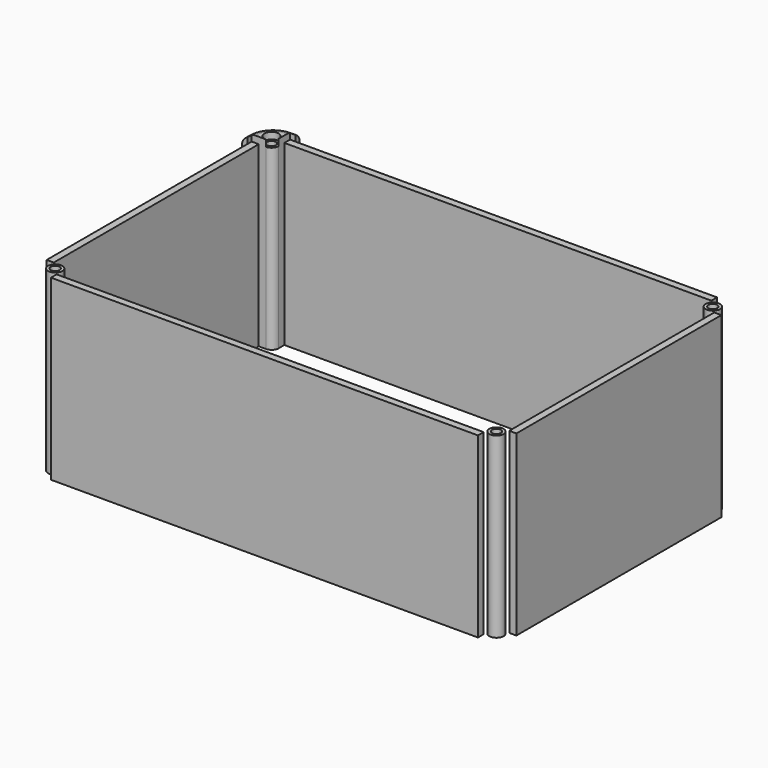
from build123d import *

# Parameters (mm, degrees)
F0_R        = 2.5
F1_DEPTH    = 100
F0_R_2      = 4
F0_W        = 240
F0_H        = 4
F0_W_2      = 4
F0_H_2      = 144
F2_DEPTH    = 103.7
F3_T1_DEPTH = 15.5
F3_T3_DEPTH = 15.5
F3_T6_ANGLE = 90


# Not quite as in the source:
# - a fillet or chamfer that OpenCascade refuses, or shapes differently, is made with other operations: its cross-section is extruded or revolved along the edge and cut away or added


with BuildPart() as f1:
    # F0 (on Top) → F1 (new body)
    with BuildSketch(Plane.XY):
        with BuildLine():
            ThreePointArc((-124, 72), (-121.1715728753, 73.1715728753), (-120, 76))
            ThreePointArc((-120, 76), (-126.8284271247, 78.8284271247), (-124, 72))
        make_face()
        with Locations((-124, 76)):
            Circle(F0_R, mode=Mode.SUBTRACT)
    extrude(amount=F1_DEPTH)


with BuildPart() as f1b:
    # F0 (on Top) → F1, piece 2 (new body)
    with BuildSketch(Plane.XY):
        with Locations((-124, -76)):
            Circle(F0_R_2)
        with Locations((-124, -76)):
            Circle(F0_R, mode=Mode.SUBTRACT)
    extrude(amount=F1_DEPTH)


with BuildPart() as f1c:
    # F0 (on Top) → F1, piece 3 (new body)
    with BuildSketch(Plane.XY):
        with Locations((124, -76)):
            Circle(F0_R_2)
        with Locations((124, -76)):
            Circle(F0_R, mode=Mode.SUBTRACT)
    extrude(amount=F1_DEPTH)


with BuildPart() as f1d:
    # F0 (on Top) → F1, piece 4 (new body)
    with BuildSketch(Plane.XY):
        with Locations((124, 76)):
            Circle(F0_R_2)
        with Locations((124, 76)):
            Circle(F0_R, mode=Mode.SUBTRACT)
    extrude(amount=F1_DEPTH)


with BuildPart() as f1e:
    # F0 (on Top) → F1, piece 5 (new body)
    with BuildSketch(Plane.XY):
        Polygon((-120, 84), (-120, 80), (120, 80), (120, 84), (-117, 84), align=None)
    extrude(amount=F1_DEPTH)


with BuildPart() as f1f:
    # F0 (on Top) → F1, piece 6 (new body)
    with BuildSketch(Plane.XY):
        Polygon((-128, -72), (-128, 72), (-132, 72), (-132, 69), (-132, -72), align=None)
    extrude(amount=F1_DEPTH)


with BuildPart() as f1g:
    # F0 (on Top) → F1, piece 7 (new body)
    with BuildSketch(Plane.XY):
        with Locations((0, -82)):
            Rectangle(F0_W, F0_H)
    extrude(amount=F1_DEPTH)


with BuildPart() as f1h:
    # F0 (on Top) → F1, piece 8 (new body)
    with BuildSketch(Plane.XY):
        with Locations((130, 0)):
            Rectangle(F0_W_2, F0_H_2)
    extrude(amount=F1_DEPTH)


with BuildPart() as f2:
    # F0 (on Top) → F2 (new body)
    with BuildSketch(Plane.XY):
        with BuildLine():
            ThreePointArc((-124, 72), (-126.8284271247, 78.8284271247), (-120, 76))
            Line((-120, 76), (-120, 80))
            Line((-120, 80), (-120, 84))
            Line((-120, 84), (-117, 84))
            Line((-117, 84), (-117, 87))
            Line((-117, 87), (-120, 87))
            ThreePointArc((-120, 87), (-130.6066017178, 82.6066017178), (-135, 72))
            Line((-135, 72), (-135, 69))
            Line((-135, 69), (-132, 69))
            Line((-132, 69), (-132, 72))
            Line((-132, 72), (-128, 72))
            Line((-128, 72), (-124, 72))
        make_face()
    extrude(amount=F2_DEPTH)

    # F3: fillet of radius 5 on 1 edges, made by hand

    # F3_s2 → F3_t1 (cut)
    with BuildSketch(Plane.YZ.offset(-120)):
        with BuildLine():
            ThreePointArc((82, 103.7), (85.5355339059, 102.2355339059), (87, 98.7))
            Line((87, 98.7), (87, 103.7))
            Line((87, 103.7), (82, 103.7))
        make_face()
    extrude(amount=F3_T1_DEPTH, mode=Mode.SUBTRACT)

    # F3_s4 → F3_t3 (cut)
    with BuildSketch(Plane.XZ.offset(-72)):
        with BuildLine():
            ThreePointArc((-135, 98.7), (-133.5355339059, 102.2355339059), (-130, 103.7))
            Line((-130, 103.7), (-135, 103.7))
            Line((-135, 103.7), (-135, 98.7))
        make_face()
    extrude(amount=F3_T3_DEPTH, mode=Mode.SUBTRACT)

    # F3_s5 → F3_t6 (revolve, cut)
    with BuildSketch(Plane.YZ.offset(-120)):
        with BuildLine():
            ThreePointArc((82, 103.7), (85.5355339059, 102.2355339059), (87, 98.7))
            Line((87, 98.7), (87, 103.7))
            Line((87, 103.7), (82, 103.7))
        make_face()
    revolve(axis=Axis((-120, 72, 103.7), (0, 0, 1)), revolution_arc=F3_T6_ANGLE, mode=Mode.SUBTRACT)


solid = Compound([f1.part, f1b.part, f1c.part, f1d.part, f1e.part, f1f.part, f1g.part, f1h.part, f2.part])
